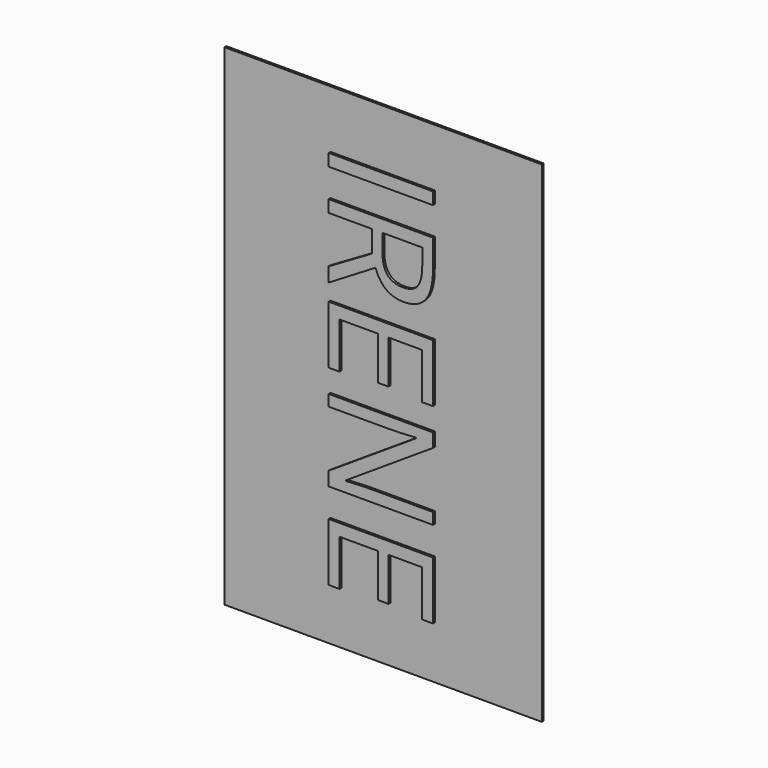
from build123d import *

# Parameters (mm, degrees)
F0_W         = 55
F0_H         = 85
F1_DEPTH     = 0.4
F2_TEXT_SIZE = 25.2907304957
F3_DEPTH     = 0.4


# Not quite as in the source:
# - Text() gives the source's letters only with a copy of the font that has no kerning and outlines rounded to 1/6400 em; it was checked with that copy


with BuildPart() as f1:
    # F0 (on Front) → F1 (new body)
    with BuildSketch(Plane.XZ):
        Rectangle(F0_W, F0_H)
    extrude(amount=F1_DEPTH)

    # F2 (on face) → F3 (join)
    with BuildSketch(Plane.XZ.offset(0.4)):
        with Locations(Location((-9.1046629784, 35), (0, 0, -90))):
            Text('IRENE', F2_TEXT_SIZE, font='Open Sans', text_align=(TextAlign.LEFT, TextAlign.BOTTOM))
    extrude(amount=F3_DEPTH)


solid = f1.part
